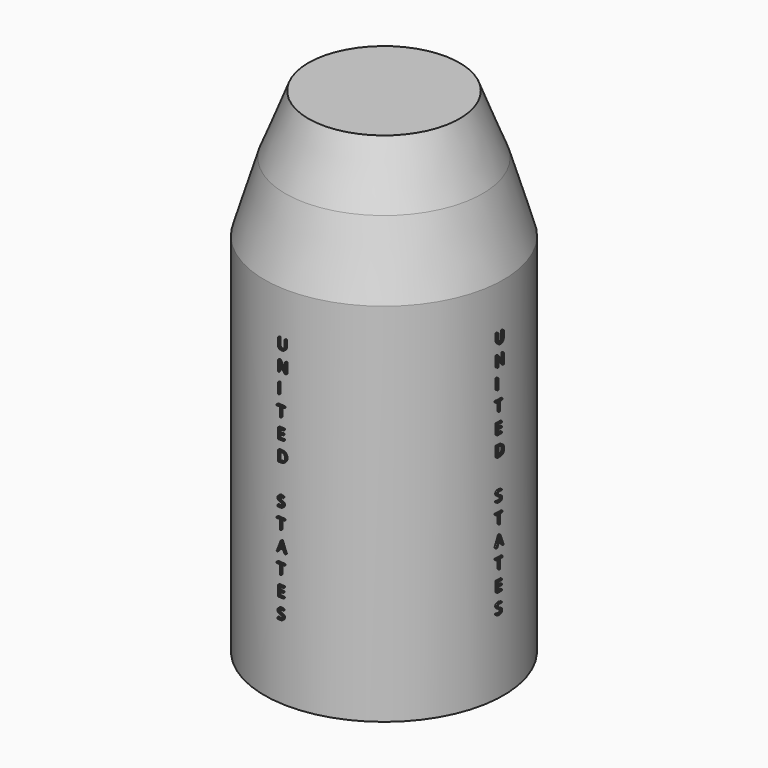
from build123d import *

# Parameters (mm, degrees)
F0_W         = 35.56
F0_H         = 108.844521417
F3_TEXT_SIZE = 4.3340441253
F4_DEPTH     = 2.9464
F5_COUNT     = 4


# Not quite as in the source:
# - Text() gives the source's letters only with a copy of the font that has no kerning and outlines rounded to 1/6400 em; it was checked with that copy


with BuildPart() as f1:
    # F0 (on Front) → F1 (revolve)
    with BuildSketch(Plane.XZ):
        with Locations((-17.78, -20.9323666032)):
            Rectangle(F0_W, F0_H)
        Polygon((-35.56, 33.4898941052), (0, 33.4898941052), (0, 53.9876818657), (-29.3300915509, 53.9876818657), align=None)
        Polygon((-29.3300915509, 53.9876818657), (0, 53.9876818657), (0, 71.3991895318), (-22.4898569286, 71.3991895318), align=None)
    revolve(axis=Axis((0, 0, 1.7531737685), (0, 0, -1)))


with BuildPart() as f4:
    # F3 (on offset) → F4 (new body)
    with BuildSketch(Plane.XZ.offset(33.02)):
        with Locations((-3.1760417106, 17.5152001902)):
            Text('U', F3_TEXT_SIZE, font='Open Sans', text_align=(TextAlign.LEFT, TextAlign.BOTTOM))
        with Locations((-3.1760417106, 11.6209001798)):
            Text('N', F3_TEXT_SIZE, font='Open Sans', text_align=(TextAlign.LEFT, TextAlign.BOTTOM))
        with Locations((-3.1760417106, 5.7266001693)):
            Text('I', F3_TEXT_SIZE, font='Open Sans', text_align=(TextAlign.LEFT, TextAlign.BOTTOM))
        with Locations((-3.1760417106, -0.1676998412)):
            Text('T', F3_TEXT_SIZE, font='Open Sans', text_align=(TextAlign.LEFT, TextAlign.BOTTOM))
        with Locations((-3.1760417106, -6.0619998516)):
            Text('E', F3_TEXT_SIZE, font='Open Sans', text_align=(TextAlign.LEFT, TextAlign.BOTTOM))
        with Locations((-3.1760417106, -11.9562998621)):
            Text('D', F3_TEXT_SIZE, font='Open Sans', text_align=(TextAlign.LEFT, TextAlign.BOTTOM))
        with Locations((-3.1760417106, -23.744899883)):
            Text('S', F3_TEXT_SIZE, font='Open Sans', text_align=(TextAlign.LEFT, TextAlign.BOTTOM))
        with Locations((-3.1760417106, -29.6391998935)):
            Text('T', F3_TEXT_SIZE, font='Open Sans', text_align=(TextAlign.LEFT, TextAlign.BOTTOM))
        with Locations((-3.1760417106, -35.533499904)):
            Text('A', F3_TEXT_SIZE, font='Open Sans', text_align=(TextAlign.LEFT, TextAlign.BOTTOM))
        with Locations((-3.1760417106, -41.4277999144)):
            Text('T', F3_TEXT_SIZE, font='Open Sans', text_align=(TextAlign.LEFT, TextAlign.BOTTOM))
        with Locations((-3.1760417106, -47.3220999249)):
            Text('E', F3_TEXT_SIZE, font='Open Sans', text_align=(TextAlign.LEFT, TextAlign.BOTTOM))
        with Locations((-3.1760417106, -53.2163999354)):
            Text('S', F3_TEXT_SIZE, font='Open Sans', text_align=(TextAlign.LEFT, TextAlign.BOTTOM))
    extrude(amount=F4_DEPTH)


with BuildPart() as f5_1:
    # F5: instance of F4
    add(f4.part.rotate(Axis((0, 0, 71.3991895318), (0, 0, -1)), 1 * 360 / F5_COUNT))


with BuildPart() as f5_2:
    # F5: instance of F4
    add(f4.part.rotate(Axis((0, 0, 71.3991895318), (0, 0, -1)), 2 * 360 / F5_COUNT))


with BuildPart() as f5_3:
    # F5: instance of F4
    add(f4.part.rotate(Axis((0, 0, 71.3991895318), (0, 0, -1)), 3 * 360 / F5_COUNT))


solid = Compound([f1.part, f4.part, f5_1.part, f5_2.part, f5_3.part])
